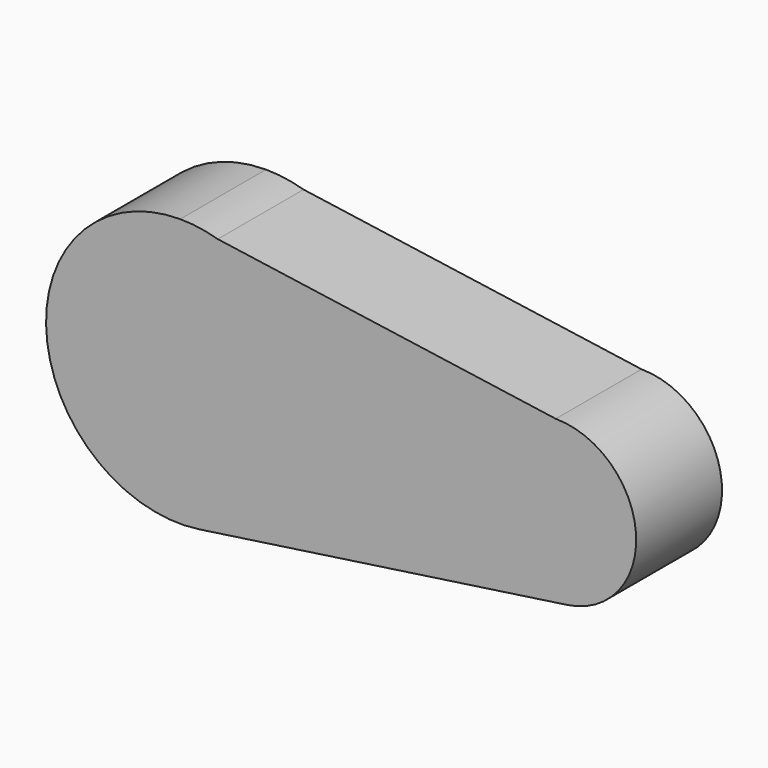
from build123d import *

# Parameters (mm, degrees)
F1_DEPTH = 50.8


# Not quite as in the source:
# - ends of sketch curves that miss each other by under 0.0002 mm in the source are joined
# - the program builds the solid bodies; features that only make, move or delete a surface that nothing else refers to are left out


with BuildPart() as f1:
    # F0 (on Front) → F1 (new body)
    with BuildSketch(Plane.XZ):
        with BuildLine():
            Line((17.78, 60.96), (0, 63.5))
            ThreePointArc((0, 63.5), (-63.3361196825, -4.5591604017), (9.0947883103, -62.845324612))
            ThreePointArc((9.0947883103, -62.845324612), (48.0092129581, -41.561586485), (63.5, 0))
            ThreePointArc((63.5, 0), (50.8, 38.1), (17.78, 60.96))
        make_face()
        with BuildLine():
            ThreePointArc((17.78, 60.96), (8.9802561211, 62.8617928475), (0, 63.5))
            Line((0, 63.5), (17.78, 60.96))
        make_face()
        with BuildLine():
            ThreePointArc((63.5, 0), (48.0092129581, -41.561586485), (9.0947883103, -62.845324612))
            Line((9.0947883103, -62.845324612), (183.2428571429, -37.7092204391))
            ThreePointArc((183.2428571429, -37.7092204391), (139.7978204656, -2.7284337331), (177.8, 38.1))
            Line((177.8, 38.1), (17.78, 60.96))
            ThreePointArc((17.78, 60.96), (50.8, 38.1), (63.5, 0))
        make_face()
        with BuildLine():
            ThreePointArc((177.8, 38.1), (139.7978204656, -2.7284337331), (183.2428571429, -37.7092204391))
            ThreePointArc((183.2428571429, -37.7092204391), (206.6008928433, -24.942304854), (215.9, 0))
            ThreePointArc((215.9, 0), (204.7407683632, 26.9407683632), (177.8, 38.1))
        make_face()
    extrude(amount=F1_DEPTH)


solid = f1.part
